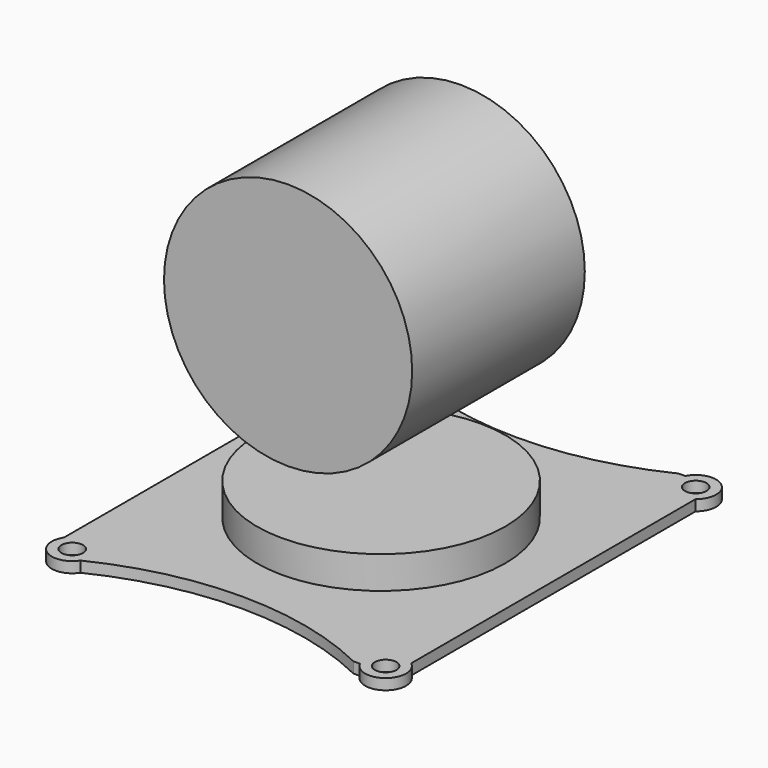
from build123d import *

# Parameters (mm, degrees)
F0_R     = 1
F0_R_2   = 11.5
F1_DEPTH = 1
F2_DEPTH = 4
F7_START = -2
F6_R     = 11.5
F7_DEPTH = 20


# Not quite as in the source:
# - the program builds the solid bodies; features that only make, move or delete a surface that nothing else refers to are left out


with BuildPart() as f1:
    # F0 (on Top) → F1 (new body)
    with BuildSketch(Plane.XY):
        with BuildLine():
            ThreePointArc((-12.7867098571, -18.8420887816), (-0.1397777075, -15.9334011427), (12.507154442, -18.8420887816))
            Line((12.507154442, -18.8420887816), (13.112995763, -18.8420887816))
            ThreePointArc((13.112995763, -18.8420887816), (16.0030328943, -19.4174459822), (15.9661910202, -16.4709237602))
            Line((15.9661910202, -16.4709237602), (15.9661910202, 16.4709237602))
            ThreePointArc((15.9661910202, 16.4709237602), (16.0030328943, 19.4174459822), (13.112995763, 18.8420887816))
            Line((13.112995763, 18.8420887816), (12.507154442, 18.8420887816))
            ThreePointArc((12.507154442, 18.8420887816), (-0.1397777075, 15.9334011427), (-12.7867098571, 18.8420887816))
            ThreePointArc((-12.7867098571, 18.8420887816), (-15.41057285, 19.3977069518), (-15.9661910202, 16.7738439589))
            Line((-15.9661910202, 16.7738439589), (-15.9661910202, -16.7738439589))
            ThreePointArc((-15.9661910202, -16.7738439589), (-15.41057285, -19.3977069518), (-12.7867098571, -18.8420887816))
        make_face()
        with Locations((-14.3764504387, -17.8079663703)):
            Circle(F0_R, mode=Mode.SUBTRACT)
        with Locations((14.791072625, -17.9591083038)):
            Circle(F0_R, mode=Mode.SUBTRACT)
        Circle(F0_R_2, mode=Mode.SUBTRACT)
        with Locations((-14.3764504387, 17.8079663703)):
            Circle(F0_R, mode=Mode.SUBTRACT)
        with Locations((14.791072625, 17.9591083038)):
            Circle(F0_R, mode=Mode.SUBTRACT)
    extrude(amount=F1_DEPTH)

    # F0 (on Top) → F2 (join)
    with BuildSketch(Plane.XY):
        Circle(F0_R_2)
    extrude(amount=F2_DEPTH)


with BuildPart() as f7:
    # F6 (on offset) → F7 (new body)
    with BuildSketch(Plane.XZ.offset(11.6).offset(F7_START)):
        with Locations((-0.9408069891, 20.2809050679)):
            Circle(F6_R)
    extrude(amount=-F7_DEPTH)


solid = Compound([f1.part, f7.part])
